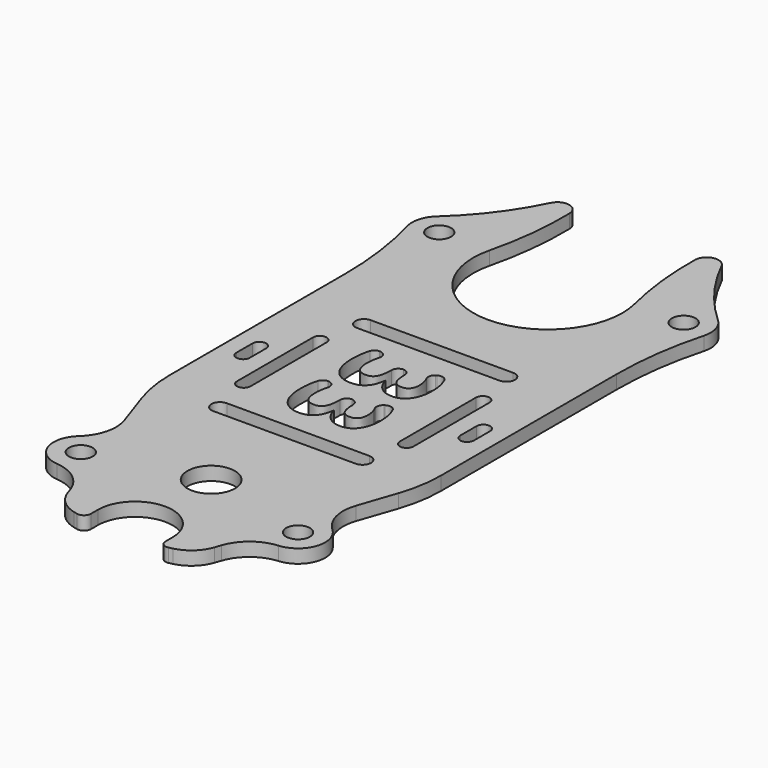
from build123d import *

# Parameters (mm, degrees)
F0_R        = 1.75
F0_R_2      = 3.5
F1_DEPTH    = 2
F2_T1_DEPTH = 2


# Not quite as in the source:
# - a fillet or chamfer that OpenCascade refuses, or shapes differently, is made with other operations: its cross-section is extruded or revolved along the edge and cut away or added


with BuildPart() as f1:
    # F0 (on Top) → F1 (new body)
    with BuildSketch(Plane.XY):
        with BuildLine():
            ThreePointArc((-12.5713700234, 50.2695594093), (-16.118909248, 44.4802706126), (-20.6903729233, 39.460049583))
            ThreePointArc((-20.6903729233, 39.460049583), (-21.8414318775, 37.6150789796), (-21.8571428571, 35.4405430733))
            ThreePointArc((-21.8571428571, 35.4405430733), (-20.4663771338, 28.6163953155), (-20, 21.6676030258))
            Line((-20, 21.6676030258), (-20, -10.6856030045))
            ThreePointArc((-20, -10.6856030045), (-19.7308995433, -13.9554047127), (-18.9308396789, -17.1372159077))
            Line((-18.9308396789, -17.1372159077), (-17.0470641697, -22.6647409918))
            ThreePointArc((-17.0470641697, -22.6647409918), (-16.9162578432, -26.0979642803), (-18.6905264293, -29.0400899451))
            ThreePointArc((-18.6905264293, -29.0400899451), (-19.7861679358, -33.2903225806), (-16.3230484377, -35.9869336221))
            ThreePointArc((-16.3230484377, -35.9869336221), (-13.1213600073, -37.2332576723), (-11.1283691906, -40.0318501842))
            Line((-11.1283691906, -40.0318501842), (-10.837240035, -40.8861046865))
            ThreePointArc((-10.837240035, -40.8861046865), (-9.4747581102, -42.9666501557), (-7.2784782144, -44.1334325108))
            ThreePointArc((-7.2784782144, -44.1334325108), (-6.9978751723, -44.1998301829), (-6.7166666667, -44.2636149343))
            ThreePointArc((-6.7166666667, -44.2636149343), (-5.8741672215, -44.067326555), (-5.5, -43.2873692912))
            Line((-5.5, -43.2873692912), (-5.5, -42))
            ThreePointArc((-5.5, -42), (0, -36.5), (5.5, -42))
            Line((5.5, -42), (5.5, -43.2873692912))
            ThreePointArc((5.5, -43.2873692912), (5.8741672215, -44.067326555), (6.7166666667, -44.2636149343))
            ThreePointArc((6.7166666667, -44.2636149343), (6.9978751723, -44.1998301829), (7.2784782144, -44.1334325108))
            ThreePointArc((7.2784782144, -44.1334325108), (9.4747581102, -42.9666501557), (10.837240035, -40.8861046865))
            Line((10.837240035, -40.8861046865), (11.1283691906, -40.0318501842))
            ThreePointArc((11.1283691906, -40.0318501842), (13.1213600073, -37.2332576723), (16.3230484377, -35.9869336221))
            ThreePointArc((16.3230484377, -35.9869336221), (19.7861679358, -33.2903225806), (18.6905264293, -29.0400899451))
            ThreePointArc((18.6905264293, -29.0400899451), (16.9162578432, -26.0979642803), (17.0470641697, -22.6647409918))
            Line((17.0470641697, -22.6647409918), (18.9308396789, -17.1372159077))
            ThreePointArc((18.9308396789, -17.1372159077), (19.7308995433, -13.9554047127), (20, -10.6856030045))
            Line((20, -10.6856030045), (20, 21.6676030258))
            ThreePointArc((20, 21.6676030258), (20.4663771338, 28.6163953155), (21.8571428571, 35.4405430733))
            ThreePointArc((21.8571428571, 35.4405430733), (21.8414318775, 37.6150789796), (20.6903729233, 39.460049583))
            ThreePointArc((20.6903729233, 39.460049583), (16.118909248, 44.4802706126), (12.5713700234, 50.2695594093))
            ThreePointArc((12.5713700234, 50.2695594093), (10.6215560146, 51.2086657952), (9.25, 49.5345900586))
            ThreePointArc((9.25, 49.5345900586), (9.5452241746, 43.0321205381), (10.6826647736, 36.6231037599))
            ThreePointArc((10.6826647736, 36.6231037599), (8.6560424375, 27.2122957253), (0, 23))
            ThreePointArc((0, 23), (-8.6560424375, 27.2122957253), (-10.6826647736, 36.6231037599))
            ThreePointArc((-10.6826647736, 36.6231037599), (-9.5452241746, 43.0321205381), (-9.25, 49.5345900586))
            ThreePointArc((-9.25, 49.5345900586), (-10.6215560146, 51.2086657952), (-12.5713700234, 50.2695594093))
        make_face()
        with Locations((-16, -32)):
            Circle(F0_R, mode=Mode.SUBTRACT)
        with BuildLine():
            Line((-17.5, -1.5), (-17.5, 1.5))
            ThreePointArc((-17.5, 1.5), (-16.5, 2.5), (-15.5, 1.5))
            Line((-15.5, 1.5), (-15.5, -1.5))
            ThreePointArc((-15.5, -1.5), (-16.5, -2.5), (-17.5, -1.5))
        make_face(mode=Mode.SUBTRACT)
        with BuildLine():
            Line((-13, -7), (-13, 7))
            ThreePointArc((-13, 7), (-12, 8), (-11, 7))
            Line((-11, 7), (-11, -7))
            ThreePointArc((-11, -7), (-12, -8), (-13, -7))
        make_face(mode=Mode.SUBTRACT)
        with BuildLine():
            add(Edge.make_bspline(
                [(5.3190104167, -7.2317708333), (4.5703125, -8.3020833333), (3.2369791667, -8.3020833333)],
                knots=[0, 0, 0, 1, 1, 1], degree=2))
            add(Edge.make_bspline(
                [(3.2369791667, -8.3020833333), (2.1223958333, -8.3020833333), (1.3411458333, -7.6263020833)],
                knots=[0, 0, 0, 1, 1, 1], degree=2))
            add(Edge.make_bspline(
                [(1.3411458333, -7.6263020833), (0.5598958333, -6.9505208333), (0.265625, -5.7291666667)],
                knots=[0, 0, 0, 1, 1, 1], degree=2))
            Line((0.265625, -5.7291666667), (0.21875, -5.7291666667))
            add(Edge.make_bspline(
                [(0.21875, -5.7291666667), (0.0390625, -7.171875), (-0.6575520833, -7.9114583333)],
                knots=[0, 0, 0, 1, 1, 1], degree=2))
            add(Edge.make_bspline(
                [(-0.6575520833, -7.9114583333), (-1.3541666667, -8.6510416667), (-2.5338541667, -8.6510416667)],
                knots=[0, 0, 0, 1, 1, 1], degree=2))
            add(Edge.make_bspline(
                [(-2.5338541667, -8.6510416667), (-4.25, -8.6510416667), (-5.20703125, -7.40625)],
                knots=[0, 0, 0, 1, 1, 1], degree=2))
            add(Edge.make_bspline(
                [(-5.20703125, -7.40625), (-6.1640625, -6.1614583333), (-6.1640625, -3.8515625)],
                knots=[0, 0, 0, 1, 1, 1], degree=2))
            add(Edge.make_bspline(
                [(-6.1640625, -3.8515625), (-6.1640625, -1.9140625), (-5.5208333333, -0.4166666667)],
                knots=[0, 0, 0, 1, 1, 1], degree=2))
            Line((-5.5208333333, -0.4166666667), (-3.3802083333, -0.4166666667))
            add(Edge.make_bspline(
                [(-3.3802083333, -0.4166666667), (-3.7291666667, -1.1067708333), (-3.94921875, -1.9375)],
                knots=[0, 0, 0, 1, 1, 1], degree=2))
            add(Edge.make_bspline(
                [(-3.94921875, -1.9375), (-4.1692708333, -2.7682291667), (-4.1692708333, -3.5807291667)],
                knots=[0, 0, 0, 1, 1, 1], degree=2))
            add(Edge.make_bspline(
                [(-4.1692708333, -3.5807291667), (-4.1692708333, -4.828125), (-3.74609375, -5.421875)],
                knots=[0, 0, 0, 1, 1, 1], degree=2))
            add(Edge.make_bspline(
                [(-3.74609375, -5.421875), (-3.3229166667, -6.015625), (-2.3854166667, -6.015625)],
                knots=[0, 0, 0, 1, 1, 1], degree=2))
            add(Edge.make_bspline(
                [(-2.3854166667, -6.015625), (-1.5494791667, -6.015625), (-1.19921875, -5.33203125)],
                knots=[0, 0, 0, 1, 1, 1], degree=2))
            add(Edge.make_bspline(
                [(-1.19921875, -5.33203125), (-0.8489583333, -4.6484375), (-0.8489583333, -3.1510416667)],
                knots=[0, 0, 0, 1, 1, 1], degree=2))
            Line((-0.8489583333, -3.1510416667), (-0.8489583333, -2.2473958333))
            Line((-0.8489583333, -2.2473958333), (1.0807291667, -2.2473958333))
            Line((1.0807291667, -2.2473958333), (1.0807291667, -3.1666666667))
            add(Edge.make_bspline(
                [(1.0807291667, -3.1666666667), (1.0807291667, -4.5494791667), (1.4427083333, -5.1888020833)],
                knots=[0, 0, 0, 1, 1, 1], degree=2))
            add(Edge.make_bspline(
                [(1.4427083333, -5.1888020833), (1.8046875, -5.828125), (2.6822916667, -5.828125)],
                knots=[0, 0, 0, 1, 1, 1], degree=2))
            add(Edge.make_bspline(
                [(2.6822916667, -5.828125), (4.0338541667, -5.828125), (4.0338541667, -4.1354166667)],
                knots=[0, 0, 0, 1, 1, 1], degree=2))
            add(Edge.make_bspline(
                [(4.0338541667, -4.1354166667), (4.0338541667, -3.5494791667), (3.8385416667, -2.9427083333)],
                knots=[0, 0, 0, 1, 1, 1], degree=2))
            add(Edge.make_bspline(
                [(3.8385416667, -2.9427083333), (3.6432291667, -2.3359375), (3.1640625, -1.5963541667)],
                knots=[0, 0, 0, 1, 1, 1], degree=2))
            Line((3.1640625, -1.5963541667), (4.8958333333, -0.4322916667))
            add(Edge.make_bspline(
                [(4.8958333333, -0.4322916667), (6.0677083333, -2.0598958333), (6.0677083333, -4.3151041667)],
                knots=[0, 0, 0, 1, 1, 1], degree=2))
            add(Edge.make_bspline(
                [(6.0677083333, -4.3151041667), (6.0677083333, -6.1614583333), (5.3190104167, -7.2317708333)],
                knots=[0, 0, 0, 1, 1, 1], degree=2))
        make_face(mode=Mode.SUBTRACT)
        with Locations((0, -28)):
            Circle(F0_R_2, mode=Mode.SUBTRACT)
        with Locations((16, -32)):
            Circle(F0_R, mode=Mode.SUBTRACT)
        with BuildLine():
            Line((10.5, -14.5), (-10.5, -14.5))
            ThreePointArc((-10.5, -14.5), (-11.75, -13.25), (-10.5, -12))
            Line((-10.5, -12), (10.5, -12))
            ThreePointArc((10.5, -12), (11.75, -13.25), (10.5, -14.5))
        make_face(mode=Mode.SUBTRACT)
        with BuildLine():
            Line((11, -7), (11, 7))
            ThreePointArc((11, 7), (12, 8), (13, 7))
            Line((13, 7), (13, -7))
            ThreePointArc((13, -7), (12, -8), (11, -7))
        make_face(mode=Mode.SUBTRACT)
        with BuildLine():
            Line((15.5, -1.5), (15.5, 1.5))
            ThreePointArc((15.5, 1.5), (16.5, 2.5), (17.5, 1.5))
            Line((17.5, 1.5), (17.5, -1.5))
            ThreePointArc((17.5, -1.5), (16.5, -2.5), (15.5, -1.5))
        make_face(mode=Mode.SUBTRACT)
        with BuildLine():
            add(Edge.make_bspline(
                [(5.3190104167, 2.28125), (4.5703125, 1.2109375), (3.2369791667, 1.2109375)],
                knots=[0, 0, 0, 1, 1, 1], degree=2))
            add(Edge.make_bspline(
                [(3.2369791667, 1.2109375), (2.1223958333, 1.2109375), (1.3411458333, 1.88671875)],
                knots=[0, 0, 0, 1, 1, 1], degree=2))
            add(Edge.make_bspline(
                [(1.3411458333, 1.88671875), (0.5598958333, 2.5625), (0.265625, 3.7838541667)],
                knots=[0, 0, 0, 1, 1, 1], degree=2))
            Line((0.265625, 3.7838541667), (0.21875, 3.7838541667))
            add(Edge.make_bspline(
                [(0.21875, 3.7838541667), (0.0390625, 2.3411458333), (-0.6575520833, 1.6015625)],
                knots=[0, 0, 0, 1, 1, 1], degree=2))
            add(Edge.make_bspline(
                [(-0.6575520833, 1.6015625), (-1.3541666667, 0.8619791667), (-2.5338541667, 0.8619791667)],
                knots=[0, 0, 0, 1, 1, 1], degree=2))
            add(Edge.make_bspline(
                [(-2.5338541667, 0.8619791667), (-4.25, 0.8619791667), (-5.20703125, 2.1067708333)],
                knots=[0, 0, 0, 1, 1, 1], degree=2))
            add(Edge.make_bspline(
                [(-5.20703125, 2.1067708333), (-6.1640625, 3.3515625), (-6.1640625, 5.6614583333)],
                knots=[0, 0, 0, 1, 1, 1], degree=2))
            add(Edge.make_bspline(
                [(-6.1640625, 5.6614583333), (-6.1640625, 7.5989583333), (-5.5208333333, 9.0963541667)],
                knots=[0, 0, 0, 1, 1, 1], degree=2))
            Line((-5.5208333333, 9.0963541667), (-3.3802083333, 9.0963541667))
            add(Edge.make_bspline(
                [(-3.3802083333, 9.0963541667), (-3.7291666667, 8.40625), (-3.94921875, 7.5755208333)],
                knots=[0, 0, 0, 1, 1, 1], degree=2))
            add(Edge.make_bspline(
                [(-3.94921875, 7.5755208333), (-4.1692708333, 6.7447916667), (-4.1692708333, 5.9322916667)],
                knots=[0, 0, 0, 1, 1, 1], degree=2))
            add(Edge.make_bspline(
                [(-4.1692708333, 5.9322916667), (-4.1692708333, 4.6848958333), (-3.74609375, 4.0911458333)],
                knots=[0, 0, 0, 1, 1, 1], degree=2))
            add(Edge.make_bspline(
                [(-3.74609375, 4.0911458333), (-3.3229166667, 3.4973958333), (-2.3854166667, 3.4973958333)],
                knots=[0, 0, 0, 1, 1, 1], degree=2))
            add(Edge.make_bspline(
                [(-2.3854166667, 3.4973958333), (-1.5494791667, 3.4973958333), (-1.19921875, 4.1809895833)],
                knots=[0, 0, 0, 1, 1, 1], degree=2))
            add(Edge.make_bspline(
                [(-1.19921875, 4.1809895833), (-0.8489583333, 4.8645833333), (-0.8489583333, 6.3619791667)],
                knots=[0, 0, 0, 1, 1, 1], degree=2))
            Line((-0.8489583333, 6.3619791667), (-0.8489583333, 7.265625))
            Line((-0.8489583333, 7.265625), (1.0807291667, 7.265625))
            Line((1.0807291667, 7.265625), (1.0807291667, 6.3463541667))
            add(Edge.make_bspline(
                [(1.0807291667, 6.3463541667), (1.0807291667, 4.9635416667), (1.4427083333, 4.32421875)],
                knots=[0, 0, 0, 1, 1, 1], degree=2))
            add(Edge.make_bspline(
                [(1.4427083333, 4.32421875), (1.8046875, 3.6848958333), (2.6822916667, 3.6848958333)],
                knots=[0, 0, 0, 1, 1, 1], degree=2))
            add(Edge.make_bspline(
                [(2.6822916667, 3.6848958333), (4.0338541667, 3.6848958333), (4.0338541667, 5.3776041667)],
                knots=[0, 0, 0, 1, 1, 1], degree=2))
            add(Edge.make_bspline(
                [(4.0338541667, 5.3776041667), (4.0338541667, 5.9635416667), (3.8385416667, 6.5703125)],
                knots=[0, 0, 0, 1, 1, 1], degree=2))
            add(Edge.make_bspline(
                [(3.8385416667, 6.5703125), (3.6432291667, 7.1770833333), (3.1640625, 7.9166666667)],
                knots=[0, 0, 0, 1, 1, 1], degree=2))
            Line((3.1640625, 7.9166666667), (4.8958333333, 9.0807291667))
            add(Edge.make_bspline(
                [(4.8958333333, 9.0807291667), (6.0677083333, 7.453125), (6.0677083333, 5.1979166667)],
                knots=[0, 0, 0, 1, 1, 1], degree=2))
            add(Edge.make_bspline(
                [(6.0677083333, 5.1979166667), (6.0677083333, 3.3515625), (5.3190104167, 2.28125)],
                knots=[0, 0, 0, 1, 1, 1], degree=2))
        make_face(mode=Mode.SUBTRACT)
        with Locations((-18, 36.5)):
            Circle(F0_R, mode=Mode.SUBTRACT)
        with BuildLine():
            Line((10.5, 12), (-10.5, 12))
            ThreePointArc((-10.5, 12), (-11.75, 13.25), (-10.5, 14.5))
            Line((-10.5, 14.5), (10.5, 14.5))
            ThreePointArc((10.5, 14.5), (11.75, 13.25), (10.5, 12))
        make_face(mode=Mode.SUBTRACT)
        with Locations((18, 36.5)):
            Circle(F0_R, mode=Mode.SUBTRACT)
    extrude(amount=F1_DEPTH)

    # F2: fillet of radius 1 on 12 edges, made by hand

    # F2_s2 → F2_t1 (join)
    with BuildSketch(Plane.XY):
        with BuildLine():
            ThreePointArc((5.4823401509, 8.0731777614), (4.843595419, 8.6204570948), (4.0129893365, 8.4877806577))
            Line((4.0129893365, 8.4877806577), (3.9571236712, 8.5708917705))
            ThreePointArc((3.9571236712, 8.5708917705), (4.3986572425, 8.8672000385), (4.839967668, 9.1638402795))
            Line((4.839967668, 9.1638402795), (4.9771020437, 9.1392426381))
            ThreePointArc((4.9771020437, 9.1392426381), (5.3001177746, 8.6415597398), (5.573409567, 8.1148285845))
            Line((5.573409567, 8.1148285845), (5.4823401509, 8.0731777614))
        make_face()
        with BuildLine():
            ThreePointArc((3.9353958823, 8.4356238546), (3.5267558643, 7.8636788331), (3.5947276057, 7.1640449185))
            Line((3.5947276057, 7.1640449185), (3.5047965874, 7.119995944))
            ThreePointArc((3.5047965874, 7.119995944), (3.3039302948, 7.4968765259), (3.0800202169, 7.8622167368))
            Line((3.0800202169, 7.8622167368), (3.1081983093, 7.9997755857))
            ThreePointArc((3.1081983093, 7.9997755857), (3.4939765733, 8.2590881932), (3.8795316916, 8.5187327736))
            Line((3.8795316916, 8.5187327736), (3.9353958823, 8.4356238546))
        make_face()
        with BuildLine():
            ThreePointArc((1.0813955663, 6.2718756487), (0.7855723775, 6.9752785605), (0.0800558835, 7.266025))
            Line((0.0800558835, 7.266025), (0.0800558835, 7.3661615685))
            ThreePointArc((0.0800558835, 7.3661615685), (0.5803925251, 7.3657615685), (1.0807291667, 7.3657615685))
            Line((1.0807291667, 7.3657615685), (1.1808657352, 7.265625))
            ThreePointArc((1.1808657352, 7.265625), (1.1808657352, 6.3463541667), (1.1815295346, 6.2725972821))
            Line((1.1815295346, 6.2725972821), (1.0813955663, 6.2718756487))
        make_face()
        with BuildLine():
            ThreePointArc((0.1516589864, 7.266025), (-0.5538546526, 6.9752813949), (-0.8496806385, 6.2718836946))
            Line((-0.8496806385, 6.2718836946), (-0.9498146009, 6.2726061326))
            ThreePointArc((-0.9498146009, 6.2726061326), (-0.9490949019, 6.3619791667), (-0.9490949019, 7.265625))
            Line((-0.9490949019, 7.265625), (-0.8489583333, 7.3657615685))
            ThreePointArc((-0.8489583333, 7.3657615685), (-0.3486496735, 7.3657615685), (0.1516589864, 7.3661615685))
            Line((0.1516589864, 7.3661615685), (0.1516589864, 7.266025))
        make_face()
        with BuildLine():
            ThreePointArc((-3.8823882856, 7.8130958508), (-4.0409586866, 8.6953409018), (-4.8424375028, 9.0967541667))
            Line((-4.8424375028, 9.0967541667), (-4.8424375028, 9.1968381664))
            ThreePointArc((-4.8424375028, 9.1968381664), (-4.1113229181, 9.1964381664), (-3.3802083333, 9.1964381664))
            Line((-3.3802083333, 9.1964381664), (-3.2908936182, 9.0511912541))
            ThreePointArc((-3.2908936182, 9.0511912541), (-3.5673911757, 8.4298441391), (-3.7863833638, 7.784814019))
            Line((-3.7863833638, 7.784814019), (-3.8823882856, 7.8130958508))
        make_face()
        with BuildLine():
            ThreePointArc((-4.8235215119, 9.0967541667), (-5.4178362512, 8.9015689774), (-5.7807035945, 8.3920254967))
            Line((-5.7807035945, 8.3920254967), (-5.8764218027, 8.4217926297))
            ThreePointArc((-5.8764218027, 8.4217926297), (-5.7538395512, 8.7821164437), (-5.6129352586, 9.1359179502))
            Line((-5.6129352586, 9.1359179502), (-5.5208333333, 9.1965941667))
            ThreePointArc((-5.5208333333, 9.1965941667), (-5.1721774226, 9.1965941667), (-4.8235215119, 9.1969941667))
            Line((-4.8235215119, 9.1969941667), (-4.8235215119, 9.0967541667))
        make_face()
        with BuildLine():
            ThreePointArc((-3.8823882856, -1.6999249825), (-4.0409586866, -0.8176799315), (-4.8424375028, -0.4162666667))
            Line((-4.8424375028, -0.4162666667), (-4.8424375028, -0.3161826669))
            ThreePointArc((-4.8424375028, -0.3161826669), (-4.1113229181, -0.3165826669), (-3.3802083333, -0.3165826669))
            Line((-3.3802083333, -0.3165826669), (-3.2908936182, -0.4618295792))
            ThreePointArc((-3.2908936182, -0.4618295792), (-3.5673911757, -1.0831766942), (-3.7863833638, -1.7282068143))
            Line((-3.7863833638, -1.7282068143), (-3.8823882856, -1.6999249825))
        make_face()
        with BuildLine():
            ThreePointArc((-4.8235215119, -0.4162666667), (-5.4178362512, -0.611451856), (-5.7807035945, -1.1209953366))
            Line((-5.7807035945, -1.1209953366), (-5.8764218027, -1.0912282036))
            ThreePointArc((-5.8764218027, -1.0912282036), (-5.7538395512, -0.7309043896), (-5.6129352586, -0.3771028831))
            Line((-5.6129352586, -0.3771028831), (-5.5208333333, -0.3164266667))
            ThreePointArc((-5.5208333333, -0.3164266667), (-5.1721774226, -0.3164266667), (-4.8235215119, -0.3160266667))
            Line((-4.8235215119, -0.3160266667), (-4.8235215119, -0.4162666667))
        make_face()
        with BuildLine():
            ThreePointArc((0.1516589864, -2.2469958333), (-0.5538546526, -2.5377394384), (-0.8496806385, -3.2411371388))
            Line((-0.8496806385, -3.2411371388), (-0.9498146009, -3.2404147008))
            ThreePointArc((-0.9498146009, -3.2404147008), (-0.9490949019, -3.1510416667), (-0.9490949019, -2.2473958333))
            Line((-0.9490949019, -2.2473958333), (-0.8489583333, -2.1472592648))
            ThreePointArc((-0.8489583333, -2.1472592648), (-0.3486496735, -2.1472592648), (0.1516589864, -2.1468592648))
            Line((0.1516589864, -2.1468592648), (0.1516589864, -2.2469958333))
        make_face()
        with BuildLine():
            ThreePointArc((1.0813955663, -3.2411451846), (0.7855723775, -2.5377422728), (0.0800558835, -2.2469958333))
            Line((0.0800558835, -2.2469958333), (0.0800558835, -2.1468592648))
            ThreePointArc((0.0800558835, -2.1468592648), (0.5803925251, -2.1472592648), (1.0807291667, -2.1472592648))
            Line((1.0807291667, -2.1472592648), (1.1808657352, -2.2473958333))
            ThreePointArc((1.1808657352, -2.2473958333), (1.1808657352, -3.1666666667), (1.1815295346, -3.2404235512))
            Line((1.1815295346, -3.2404235512), (1.0813955663, -3.2411451846))
        make_face()
        with BuildLine():
            ThreePointArc((3.9353958823, -1.0773969787), (3.5267558643, -1.6493420003), (3.5947276057, -2.3489759148))
            Line((3.5947276057, -2.3489759148), (3.5047965874, -2.3930248894))
            ThreePointArc((3.5047965874, -2.3930248894), (3.3039302948, -2.0161443075), (3.0800202169, -1.6508040966))
            Line((3.0800202169, -1.6508040966), (3.1081983093, -1.5132452476))
            ThreePointArc((3.1081983093, -1.5132452476), (3.4939765733, -1.2539326401), (3.8795316916, -0.9942880597))
            Line((3.8795316916, -0.9942880597), (3.9353958823, -1.0773969787))
        make_face()
        with BuildLine():
            ThreePointArc((4.0129893365, -1.0252401757), (4.843595419, -0.8925637385), (5.4823401509, -1.439843072))
            Line((5.4823401509, -1.439843072), (5.573409567, -1.3981922488))
            ThreePointArc((5.573409567, -1.3981922488), (5.3001177746, -0.8714610935), (4.9771020437, -0.3737781952))
            Line((4.9771020437, -0.3737781952), (4.839967668, -0.3491805539))
            ThreePointArc((4.839967668, -0.3491805539), (4.3986572425, -0.6458207948), (3.9571236712, -0.9421290629))
            Line((3.9571236712, -0.9421290629), (4.0129893365, -1.0252401757))
        make_face()
    extrude(amount=F2_T1_DEPTH)


solid = f1.part
